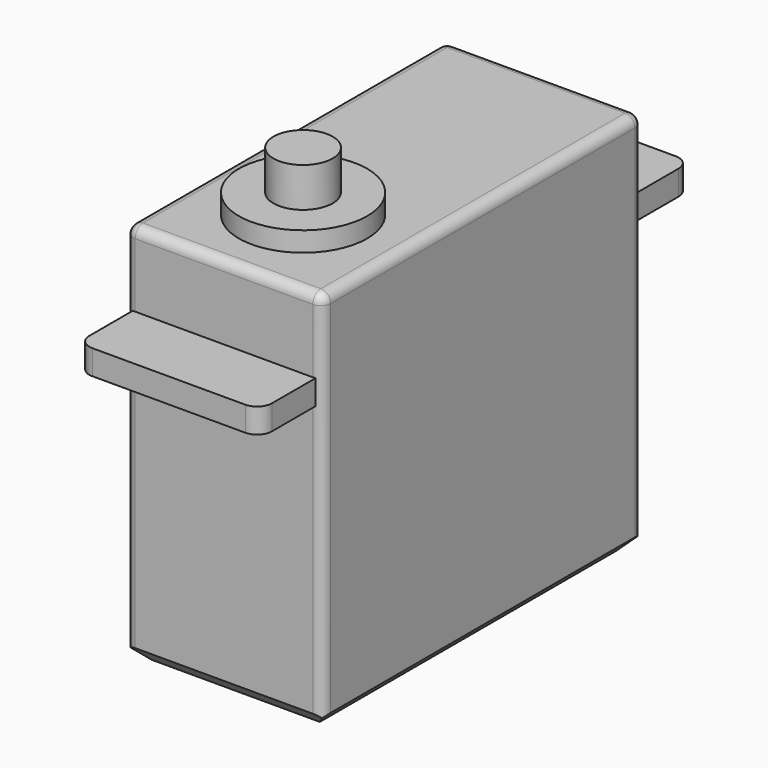
from build123d import *

# Parameters (mm, degrees)
F0_W          = 0.75
F0_H          = 40.5
F0_W_2        = 18.5
F1_DEPTH      = 29
F1_DEPTH_BACK = 10
F2_DEPTH      = 2.5
F3_R          = 6.5
F3_R_2        = 3
F4_DEPTH      = 2
F5_DEPTH      = 6
F6_SIZE       = 1.5
F7_T1_DEPTH   = 38.5
F7_T3_DEPTH   = 18
F7_S7_W       = 1
F7_S7_H       = 1
F7_T8_DEPTH   = 1
F7_S13_W      = 1
F7_S13_H      = 1
F7_T14_DEPTH  = 1
F7_S19_W      = 1
F7_S19_H      = 1
F7_T20_DEPTH  = 1
F7_S25_W      = 1
F7_S25_H      = 1
F7_T26_DEPTH  = 1
F7_T32_DEPTH  = 39
F7_T38_DEPTH  = 39
F7_T44_DEPTH  = 39
F7_T51_DEPTH  = 39
F7_T57_DEPTH  = 39
F7_T63_DEPTH  = 39
F7_T69_DEPTH  = 39
F7_T75_DEPTH  = 39
F7_T82_DEPTH  = 39
F7_T88_DEPTH  = 39
F7_T94_DEPTH  = 39
F7_T100_DEPTH = 39
F7_T106_DEPTH = 39
F7_T113_DEPTH = 39
F7_T119_DEPTH = 39
F7_T125_DEPTH = 39
F7_T131_DEPTH = 39
F7_T137_DEPTH = 39
F7_T144_DEPTH = 39
F7_T150_DEPTH = 39


# Not quite as in the source:
# - a fillet or chamfer that OpenCascade refuses, or shapes differently, is made with other operations: its cross-section is extruded or revolved along the edge and cut away or added


with BuildPart() as f1:
    # F0 (on Top) → F1 (new body, two sides)
    with BuildSketch(Plane.XY) as f1_sk:
        with Locations((9.625, 0)):
            Rectangle(F0_W, F0_H)
        Rectangle(F0_W_2, F0_H)
        with Locations((-9.625, 0)):
            Rectangle(F0_W, F0_H)
    extrude(amount=-F1_DEPTH)
    extrude(f1_sk.sketch, amount=F1_DEPTH_BACK)

    # F0 (on Top) → F2 (join)
    with BuildSketch(Plane.XY):
        with BuildLine():
            Line((9.25, -25.75), (9.25, -20.25))
            Line((9.25, -20.25), (-9.25, -20.25))
            Line((-9.25, -20.25), (-9.25, -25.75))
            ThreePointArc((-9.25, -25.75), (-8.8106601718, -26.8106601718), (-7.75, -27.25))
            Line((-7.75, -27.25), (7.75, -27.25))
            ThreePointArc((7.75, -27.25), (8.8106601718, -26.8106601718), (9.25, -25.75))
        make_face()
        with BuildLine():
            Line((-9.25, 20.25), (9.25, 20.25))
            Line((9.25, 20.25), (9.25, 25.75))
            ThreePointArc((9.25, 25.75), (8.8106601718, 26.8106601718), (7.75, 27.25))
            Line((7.75, 27.25), (-7.75, 27.25))
            ThreePointArc((-7.75, 27.25), (-8.8106601718, 26.8106601718), (-9.25, 25.75))
            Line((-9.25, 25.75), (-9.25, 20.25))
        make_face()
    extrude(amount=F2_DEPTH)

    # F3 (on face) → F4 (join)
    with BuildSketch(Plane.XY.offset(10)):
        with Locations((0, -10.25)):
            Circle(F3_R)
        with Locations((0, -10.25)):
            Circle(F3_R_2, mode=Mode.SUBTRACT)
    extrude(amount=F4_DEPTH)

    # F3 (on face) → F5 (join)
    with BuildSketch(Plane.XY.offset(10)):
        with Locations((0, -10.25)):
            Circle(F3_R_2)
    extrude(amount=F5_DEPTH)

    # F6
    f6_edges = [f1.edges().sort_by_distance(p)[0] for p in [
        (10, 0, -29),
        (0, 20.25, -29),
        (-10, 0, -29),
        (0, -20.25, -29),
    ]]
    chamfer(f6_edges, length=F6_SIZE)

    # F7: fillet of radius 1 on 8 edges, made by hand

    # F7_s2 → F7_t1 (cut)
    with BuildSketch(Plane.XZ.offset(-19.25)):
        with BuildLine():
            ThreePointArc((-9, 10), (-9.7071067812, 9.7071067812), (-10, 9))
            Line((-10, 9), (-10, 10))
            Line((-10, 10), (-9, 10))
        make_face()
        with BuildLine():
            ThreePointArc((10, 9), (9.7071067812, 9.7071067812), (9, 10))
            Line((9, 10), (10, 10))
            Line((10, 10), (10, 9))
        make_face()
    extrude(amount=F7_T1_DEPTH, mode=Mode.SUBTRACT)

    # F7_s4 → F7_t3 (cut)
    with BuildSketch(Plane.YZ.offset(-9)):
        with BuildLine():
            ThreePointArc((20.25, 9), (19.9571067812, 9.7071067812), (19.25, 10))
            Line((19.25, 10), (20.25, 10))
            Line((20.25, 10), (20.25, 9))
        make_face()
        with BuildLine():
            ThreePointArc((-19.25, 10), (-19.9571067812, 9.7071067812), (-20.25, 9))
            Line((-20.25, 9), (-20.25, 10))
            Line((-20.25, 10), (-19.25, 10))
        make_face()
    extrude(amount=F7_T3_DEPTH, mode=Mode.SUBTRACT)


with BuildPart() as f7_tool6:
    # F7_s7 → F7_t8 (new body)
    with BuildSketch(Plane.XZ.offset(-19.25)):
        with Locations((-9.5, 9.5)):
            Rectangle(F7_S7_W, F7_S7_H)
    extrude(amount=-F7_T8_DEPTH)

    # F7_s9 → F7_t10 (revolve, cut)
    with BuildSketch(Plane(origin=(-9, 19.25, 9), x_dir=(0.7071067812, 0, -0.7071067812), z_dir=(0.7071067812, 0, 0.7071067812))):
        with BuildLine():
            ThreePointArc((0, -1), (1, 0), (0, 1))
            Line((0, 1), (0, -1))
        make_face()
    revolve(axis=Axis((-9, 19.25, 9), (0, 1, 0)), mode=Mode.SUBTRACT)


with BuildPart() as f1_1:
    add(f1.part)

    # F7_t5: cut F7_tool6
    add(f7_tool6.part, mode=Mode.SUBTRACT)


with BuildPart() as f7_tool12:
    # F7_s13 → F7_t14 (new body)
    with BuildSketch(Plane.XY.offset(9)):
        with Locations((-9.5, -19.75)):
            Rectangle(F7_S13_W, F7_S13_H)
    extrude(amount=F7_T14_DEPTH)

    # F7_s15 → F7_t16 (revolve, cut)
    with BuildSketch(Plane(origin=(-9, -19.25, 9), x_dir=(0.7071067812, 0.7071067812, 0), z_dir=(0.7071067812, -0.7071067812, 0))):
        with BuildLine():
            ThreePointArc((0, -1), (1, 0), (0, 1))
            Line((0, 1), (0, -1))
        make_face()
    revolve(axis=Axis((-9, -19.25, 9), (0, 0, 1)), mode=Mode.SUBTRACT)


with BuildPart() as f1_2:
    add(f1_1.part)

    # F7_t11: cut F7_tool12
    add(f7_tool12.part, mode=Mode.SUBTRACT)


with BuildPart() as f7_tool18:
    # F7_s19 → F7_t20 (new body)
    with BuildSketch(Plane.YZ.offset(9)):
        with Locations((19.75, 9.5)):
            Rectangle(F7_S19_W, F7_S19_H)
    extrude(amount=F7_T20_DEPTH)

    # F7_s21 → F7_t22 (revolve, cut)
    with BuildSketch(Plane(origin=(9, 19.25, 9), x_dir=(0, -0.7071067812, -0.7071067812), z_dir=(0, -0.7071067812, 0.7071067812))):
        with BuildLine():
            ThreePointArc((0, -1), (1, 0), (0, 1))
            Line((0, 1), (0, -1))
        make_face()
    revolve(axis=Axis((9, 19.25, 9), (1, 0, 0)), mode=Mode.SUBTRACT)


with BuildPart() as f1_3:
    add(f1_2.part)

    # F7_t17: cut F7_tool18
    add(f7_tool18.part, mode=Mode.SUBTRACT)


with BuildPart() as f7_tool24:
    # F7_s25 → F7_t26 (new body)
    with BuildSketch(Plane.YZ.offset(9)):
        with Locations((-19.75, 9.5)):
            Rectangle(F7_S25_W, F7_S25_H)
    extrude(amount=F7_T26_DEPTH)

    # F7_s27 → F7_t28 (revolve, cut)
    with BuildSketch(Plane(origin=(9, -19.25, 9), x_dir=(0, 0.7071067812, -0.7071067812), z_dir=(0, -0.7071067812, -0.7071067812))):
        with BuildLine():
            ThreePointArc((0, -1), (1, 0), (0, 1))
            Line((0, 1), (0, -1))
        make_face()
    revolve(axis=Axis((9, -19.25, 9), (1, 0, 0)), mode=Mode.SUBTRACT)


with BuildPart() as f1_4:
    add(f1_3.part)

    # F7_t23: cut F7_tool24
    add(f7_tool24.part, mode=Mode.SUBTRACT)


with BuildPart() as f7_tool30:
    # F7_s31 → F7_t32 (new body)
    with BuildSketch(Plane.XY.offset(-30)):
        with BuildLine():
            ThreePointArc((10, 19.25), (9.7071067812, 19.9571067812), (9, 20.25))
            Line((9, 20.25), (10, 20.25))
            Line((10, 20.25), (10, 19.25))
        make_face()
    extrude(amount=F7_T32_DEPTH)

    split(bisect_by=Plane.YZ.offset(9.25), keep=Keep.TOP)

    split(bisect_by=Plane.XY, keep=Keep.BOTTOM)


with BuildPart() as f1_5:
    add(f1_4.part)

    # F7_t29: cut F7_tool30
    add(f7_tool30.part, mode=Mode.SUBTRACT)


with BuildPart() as f7_tool36:
    # F7_s37 → F7_t38 (new body)
    with BuildSketch(Plane.XY.offset(-30)):
        with BuildLine():
            ThreePointArc((10, 19.25), (9.7071067812, 19.9571067812), (9, 20.25))
            Line((9, 20.25), (10, 20.25))
            Line((10, 20.25), (10, 19.25))
        make_face()
    extrude(amount=F7_T38_DEPTH)

    split(bisect_by=Plane.YZ.offset(9.25), keep=Keep.BOTTOM)

    split(bisect_by=Plane.XY, keep=Keep.BOTTOM)


with BuildPart() as f1_6:
    add(f1_5.part)

    # F7_t35: cut F7_tool36
    add(f7_tool36.part, mode=Mode.SUBTRACT)


with BuildPart() as f7_tool42:
    # F7_s43 → F7_t44 (new body)
    with BuildSketch(Plane.XY.offset(-30)):
        with BuildLine():
            ThreePointArc((10, 19.25), (9.7071067812, 19.9571067812), (9, 20.25))
            Line((9, 20.25), (10, 20.25))
            Line((10, 20.25), (10, 19.25))
        make_face()
    extrude(amount=F7_T44_DEPTH)

    split(bisect_by=Plane.XY.offset(2.5), keep=Keep.BOTTOM)

    split(bisect_by=Plane.YZ.offset(9.25), keep=Keep.TOP)

    split(bisect_by=Plane.XY, keep=Keep.TOP)


with BuildPart() as f1_7:
    add(f1_6.part)

    # F7_t41: cut F7_tool42
    add(f7_tool42.part, mode=Mode.SUBTRACT)


with BuildPart() as f7_tool49:
    # F7_s50 → F7_t51 (new body)
    with BuildSketch(Plane.XY.offset(-30)):
        with BuildLine():
            ThreePointArc((10, 19.25), (9.7071067812, 19.9571067812), (9, 20.25))
            Line((9, 20.25), (10, 20.25))
            Line((10, 20.25), (10, 19.25))
        make_face()
    extrude(amount=F7_T51_DEPTH)

    split(bisect_by=Plane.XY.offset(2.5), keep=Keep.TOP)

    split(bisect_by=Plane.YZ.offset(9.25), keep=Keep.TOP)


with BuildPart() as f1_8:
    add(f1_7.part)

    # F7_t48: cut F7_tool49
    add(f7_tool49.part, mode=Mode.SUBTRACT)


with BuildPart() as f7_tool55:
    # F7_s56 → F7_t57 (new body)
    with BuildSketch(Plane.XY.offset(-30)):
        with BuildLine():
            ThreePointArc((10, 19.25), (9.7071067812, 19.9571067812), (9, 20.25))
            Line((9, 20.25), (10, 20.25))
            Line((10, 20.25), (10, 19.25))
        make_face()
    extrude(amount=F7_T57_DEPTH)

    split(bisect_by=Plane.XY.offset(2.5), keep=Keep.TOP)

    split(bisect_by=Plane.YZ.offset(9.25), keep=Keep.BOTTOM)


with BuildPart() as f1_9:
    add(f1_8.part)

    # F7_t54: cut F7_tool55
    add(f7_tool55.part, mode=Mode.SUBTRACT)


with BuildPart() as f7_tool61:
    # F7_s62 → F7_t63 (new body)
    with BuildSketch(Plane.XY.offset(9)):
        with BuildLine():
            ThreePointArc((-9, -20.25), (-9.7071067812, -19.9571067812), (-10, -19.25))
            Line((-10, -19.25), (-10, -20.25))
            Line((-10, -20.25), (-9, -20.25))
        make_face()
    extrude(amount=-F7_T63_DEPTH)

    split(bisect_by=Plane.XY.offset(2.5), keep=Keep.TOP)

    split(bisect_by=Plane.YZ.offset(-9.25), keep=Keep.TOP)


with BuildPart() as f1_10:
    add(f1_9.part)

    # F7_t60: cut F7_tool61
    add(f7_tool61.part, mode=Mode.SUBTRACT)


with BuildPart() as f7_tool67:
    # F7_s68 → F7_t69 (new body)
    with BuildSketch(Plane.XY.offset(9)):
        with BuildLine():
            ThreePointArc((-9, -20.25), (-9.7071067812, -19.9571067812), (-10, -19.25))
            Line((-10, -19.25), (-10, -20.25))
            Line((-10, -20.25), (-9, -20.25))
        make_face()
    extrude(amount=-F7_T69_DEPTH)

    split(bisect_by=Plane.XY.offset(2.5), keep=Keep.TOP)

    split(bisect_by=Plane.YZ.offset(-9.25), keep=Keep.BOTTOM)


with BuildPart() as f1_11:
    add(f1_10.part)

    # F7_t66: cut F7_tool67
    add(f7_tool67.part, mode=Mode.SUBTRACT)


with BuildPart() as f7_tool73:
    # F7_s74 → F7_t75 (new body)
    with BuildSketch(Plane.XY.offset(9)):
        with BuildLine():
            ThreePointArc((-9, -20.25), (-9.7071067812, -19.9571067812), (-10, -19.25))
            Line((-10, -19.25), (-10, -20.25))
            Line((-10, -20.25), (-9, -20.25))
        make_face()
    extrude(amount=-F7_T75_DEPTH)

    split(bisect_by=Plane.XY.offset(2.5), keep=Keep.BOTTOM)

    split(bisect_by=Plane.YZ.offset(-9.25), keep=Keep.BOTTOM)

    split(bisect_by=Plane.XY, keep=Keep.TOP)


with BuildPart() as f1_12:
    add(f1_11.part)

    # F7_t72: cut F7_tool73
    add(f7_tool73.part, mode=Mode.SUBTRACT)


with BuildPart() as f7_tool80:
    # F7_s81 → F7_t82 (new body)
    with BuildSketch(Plane.XY.offset(9)):
        with BuildLine():
            ThreePointArc((-9, -20.25), (-9.7071067812, -19.9571067812), (-10, -19.25))
            Line((-10, -19.25), (-10, -20.25))
            Line((-10, -20.25), (-9, -20.25))
        make_face()
    extrude(amount=-F7_T82_DEPTH)

    split(bisect_by=Plane.YZ.offset(-9.25), keep=Keep.TOP)

    split(bisect_by=Plane.XY, keep=Keep.BOTTOM)


with BuildPart() as f1_13:
    add(f1_12.part)

    # F7_t79: cut F7_tool80
    add(f7_tool80.part, mode=Mode.SUBTRACT)


with BuildPart() as f7_tool86:
    # F7_s87 → F7_t88 (new body)
    with BuildSketch(Plane.XY.offset(9)):
        with BuildLine():
            ThreePointArc((-9, -20.25), (-9.7071067812, -19.9571067812), (-10, -19.25))
            Line((-10, -19.25), (-10, -20.25))
            Line((-10, -20.25), (-9, -20.25))
        make_face()
    extrude(amount=-F7_T88_DEPTH)

    split(bisect_by=Plane.YZ.offset(-9.25), keep=Keep.BOTTOM)

    split(bisect_by=Plane.XY, keep=Keep.BOTTOM)


with BuildPart() as f1_14:
    add(f1_13.part)

    # F7_t85: cut F7_tool86
    add(f7_tool86.part, mode=Mode.SUBTRACT)


with BuildPart() as f7_tool92:
    # F7_s93 → F7_t94 (new body)
    with BuildSketch(Plane.XY.offset(9)):
        with BuildLine():
            ThreePointArc((10, -19.25), (9.7071067812, -19.9571067812), (9, -20.25))
            Line((9, -20.25), (10, -20.25))
            Line((10, -20.25), (10, -19.25))
        make_face()
    extrude(amount=-F7_T94_DEPTH)

    split(bisect_by=Plane.YZ.offset(9.25), keep=Keep.TOP)

    split(bisect_by=Plane.XY.offset(2.5), keep=Keep.TOP)


with BuildPart() as f1_15:
    add(f1_14.part)

    # F7_t91: cut F7_tool92
    add(f7_tool92.part, mode=Mode.SUBTRACT)


with BuildPart() as f7_tool98:
    # F7_s99 → F7_t100 (new body)
    with BuildSketch(Plane.XY.offset(9)):
        with BuildLine():
            ThreePointArc((10, -19.25), (9.7071067812, -19.9571067812), (9, -20.25))
            Line((9, -20.25), (10, -20.25))
            Line((10, -20.25), (10, -19.25))
        make_face()
    extrude(amount=-F7_T100_DEPTH)

    split(bisect_by=Plane.YZ.offset(9.25), keep=Keep.BOTTOM)

    split(bisect_by=Plane.XY.offset(2.5), keep=Keep.TOP)


with BuildPart() as f1_16:
    add(f1_15.part)

    # F7_t97: cut F7_tool98
    add(f7_tool98.part, mode=Mode.SUBTRACT)


with BuildPart() as f7_tool104:
    # F7_s105 → F7_t106 (new body)
    with BuildSketch(Plane.XY.offset(9)):
        with BuildLine():
            ThreePointArc((10, -19.25), (9.7071067812, -19.9571067812), (9, -20.25))
            Line((9, -20.25), (10, -20.25))
            Line((10, -20.25), (10, -19.25))
        make_face()
    extrude(amount=-F7_T106_DEPTH)

    split(bisect_by=Plane.YZ.offset(9.25), keep=Keep.TOP)

    split(bisect_by=Plane.XY.offset(2.5), keep=Keep.BOTTOM)

    split(bisect_by=Plane.XY, keep=Keep.TOP)


with BuildPart() as f1_17:
    add(f1_16.part)

    # F7_t103: cut F7_tool104
    add(f7_tool104.part, mode=Mode.SUBTRACT)


with BuildPart() as f7_tool111:
    # F7_s112 → F7_t113 (new body)
    with BuildSketch(Plane.XY.offset(9)):
        with BuildLine():
            ThreePointArc((10, -19.25), (9.7071067812, -19.9571067812), (9, -20.25))
            Line((9, -20.25), (10, -20.25))
            Line((10, -20.25), (10, -19.25))
        make_face()
    extrude(amount=-F7_T113_DEPTH)

    split(bisect_by=Plane.YZ.offset(9.25), keep=Keep.TOP)

    split(bisect_by=Plane.XY, keep=Keep.BOTTOM)


with BuildPart() as f1_18:
    add(f1_17.part)

    # F7_t110: cut F7_tool111
    add(f7_tool111.part, mode=Mode.SUBTRACT)


with BuildPart() as f7_tool117:
    # F7_s118 → F7_t119 (new body)
    with BuildSketch(Plane.XY.offset(9)):
        with BuildLine():
            ThreePointArc((10, -19.25), (9.7071067812, -19.9571067812), (9, -20.25))
            Line((9, -20.25), (10, -20.25))
            Line((10, -20.25), (10, -19.25))
        make_face()
    extrude(amount=-F7_T119_DEPTH)

    split(bisect_by=Plane.YZ.offset(9.25), keep=Keep.BOTTOM)

    split(bisect_by=Plane.XY, keep=Keep.BOTTOM)


with BuildPart() as f1_19:
    add(f1_18.part)

    # F7_t116: cut F7_tool117
    add(f7_tool117.part, mode=Mode.SUBTRACT)


with BuildPart() as f7_tool123:
    # F7_s124 → F7_t125 (new body)
    with BuildSketch(Plane.XY.offset(-30)):
        with BuildLine():
            ThreePointArc((-9, 20.25), (-9.7071067812, 19.9571067812), (-10, 19.25))
            Line((-10, 19.25), (-10, 20.25))
            Line((-10, 20.25), (-9, 20.25))
        make_face()
    extrude(amount=F7_T125_DEPTH)

    split(bisect_by=Plane.YZ.offset(-9.25), keep=Keep.TOP)

    split(bisect_by=Plane.XY, keep=Keep.BOTTOM)


with BuildPart() as f1_20:
    add(f1_19.part)

    # F7_t122: cut F7_tool123
    add(f7_tool123.part, mode=Mode.SUBTRACT)


with BuildPart() as f7_tool129:
    # F7_s130 → F7_t131 (new body)
    with BuildSketch(Plane.XY.offset(-30)):
        with BuildLine():
            ThreePointArc((-9, 20.25), (-9.7071067812, 19.9571067812), (-10, 19.25))
            Line((-10, 19.25), (-10, 20.25))
            Line((-10, 20.25), (-9, 20.25))
        make_face()
    extrude(amount=F7_T131_DEPTH)

    split(bisect_by=Plane.YZ.offset(-9.25), keep=Keep.BOTTOM)

    split(bisect_by=Plane.XY, keep=Keep.BOTTOM)


with BuildPart() as f1_21:
    add(f1_20.part)

    # F7_t128: cut F7_tool129
    add(f7_tool129.part, mode=Mode.SUBTRACT)


with BuildPart() as f7_tool135:
    # F7_s136 → F7_t137 (new body)
    with BuildSketch(Plane.XY.offset(-30)):
        with BuildLine():
            ThreePointArc((-9, 20.25), (-9.7071067812, 19.9571067812), (-10, 19.25))
            Line((-10, 19.25), (-10, 20.25))
            Line((-10, 20.25), (-9, 20.25))
        make_face()
    extrude(amount=F7_T137_DEPTH)

    split(bisect_by=Plane.YZ.offset(-9.25), keep=Keep.BOTTOM)

    split(bisect_by=Plane.XY.offset(2.5), keep=Keep.BOTTOM)

    split(bisect_by=Plane.XY, keep=Keep.TOP)


with BuildPart() as f1_22:
    add(f1_21.part)

    # F7_t134: cut F7_tool135
    add(f7_tool135.part, mode=Mode.SUBTRACT)


with BuildPart() as f7_tool142:
    # F7_s143 → F7_t144 (new body)
    with BuildSketch(Plane.XY.offset(-30)):
        with BuildLine():
            ThreePointArc((-9, 20.25), (-9.7071067812, 19.9571067812), (-10, 19.25))
            Line((-10, 19.25), (-10, 20.25))
            Line((-10, 20.25), (-9, 20.25))
        make_face()
    extrude(amount=F7_T144_DEPTH)

    split(bisect_by=Plane.YZ.offset(-9.25), keep=Keep.TOP)

    split(bisect_by=Plane.XY.offset(2.5), keep=Keep.TOP)


with BuildPart() as f1_23:
    add(f1_22.part)

    # F7_t141: cut F7_tool142
    add(f7_tool142.part, mode=Mode.SUBTRACT)


with BuildPart() as f7_tool148:
    # F7_s149 → F7_t150 (new body)
    with BuildSketch(Plane.XY.offset(-30)):
        with BuildLine():
            ThreePointArc((-9, 20.25), (-9.7071067812, 19.9571067812), (-10, 19.25))
            Line((-10, 19.25), (-10, 20.25))
            Line((-10, 20.25), (-9, 20.25))
        make_face()
    extrude(amount=F7_T150_DEPTH)

    split(bisect_by=Plane.YZ.offset(-9.25), keep=Keep.BOTTOM)

    split(bisect_by=Plane.XY.offset(2.5), keep=Keep.TOP)


with BuildPart() as f1_24:
    add(f1_23.part)

    # F7_t147: cut F7_tool148
    add(f7_tool148.part, mode=Mode.SUBTRACT)


solid = f1_24.part
